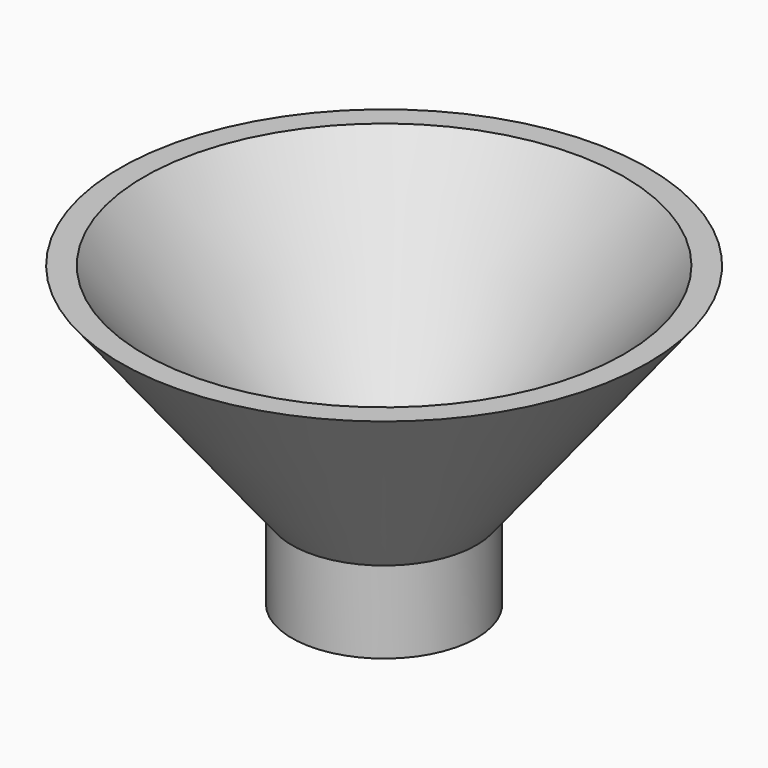
from build123d import *

# Parameters (mm, degrees)
F4_R     = 15.875
F5_DEPTH = 76.2


# Not quite as in the source:
# - a feature of the source that left no trace in its solid (it failed there, or was rolled back) is left out


with BuildPart() as f1:
    # F0 (on Front) → F1 (revolve)
    with BuildSketch(Plane.XZ):
        Polygon((0, -22.6070340723), (0, 0), (47.3772140821, 59.6811493339), (40.7688170671, 59.6811493339), (-6.0150707141, 0), (-25.4921261221, 0), (-25.4921261221, -22.6070340723), align=None)
    revolve(axis=Axis((-25.4921261221, 0, -11.3035170361), (0, 0, -1)))

    # F4 (on face) → F5 (cut)
    with BuildSketch(Plane.XY):
        with Locations((-25.4921261221, 0)):
            Circle(F4_R)
    extrude(amount=-F5_DEPTH, mode=Mode.SUBTRACT)


solid = f1.part
